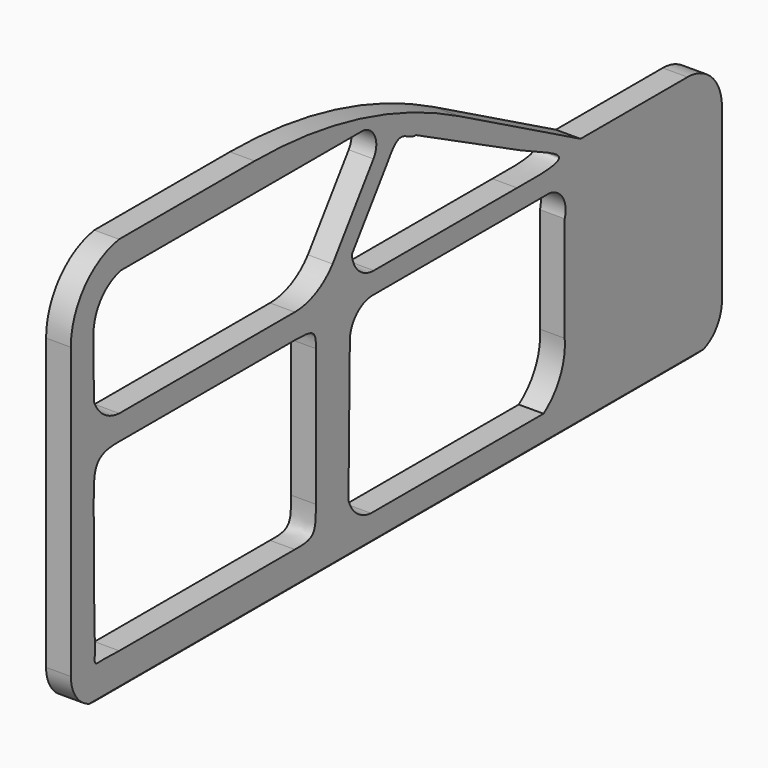
from build123d import *

# Parameters (mm, degrees)
F0_W     = 356.8245768547
F0_H     = 505.1945460796
F1_DEPTH = 50
F2_R     = 1088.3972766598
F3_R     = 86.9116882454
F4_SIZE  = 5
F5_R     = 72.4264068712


with BuildPart() as f1:
    # F0 (on Right) → F1 (new body)
    with BuildSketch(Plane.YZ):
        with BuildLine():
            Line((-202.2370483146, 445.1378583908), (-818.7412619591, 445.1378583908))
            ThreePointArc((-818.7412619591, 445.1378583908), (-905.8236422374, 396.3429239553), (-940.366268158, 302.6888072491))
            Line((-940.366268158, 302.6888072491), (-940.366268158, -354.9621416092))
            Line((-940.366268158, -354.9621416092), (345.9845781326, -354.9621416092))
            Line((345.9845781326, -354.9621416092), (345.9845781326, 150.2324044704))
            Line((345.9845781326, 150.2324044704), (-202.2370483146, 445.1378583908))
        make_face()
        with BuildLine():
            Line((-375.1508891582, -286.562114954), (-818.0344700813, -286.562114954))
            add(Edge.make_bspline(
                [(-881.003574872, -213.6291732903), (-872.4157214165, -310.1377487183), (-905.2422046661, -279.6560525894), (-818.0344700813, -286.562114954)],
                knots=[0, 0, 0, 0, 96.3551873946, 96.3551873946, 96.3551873946, 96.3551873946], degree=3))
            Line((-881.003574872, -213.6291732903), (-882.7309639931, 0))
            add(Edge.make_bspline(
                [(-882.7309639931, 0), (-883.1830024719, 63.9973655343), (-881.788790226, 86.3044932485), (-818.0344700813, 85.4378938675)],
                knots=[0, 0, 0, 0, 107.1693521161, 107.1693521161, 107.1693521161, 107.1693521161], degree=3))
            Line((-818.0344700813, 85.4378938675), (-375.1508891582, 85.4378938675))
            add(Edge.make_bspline(
                [(-375.1508891582, 85.4378938675), (-324.9171972275, 85.5383649468), (-321.6931819916, 79.6764940023), (-321.9781610433, 48.8521754742)],
                knots=[0, 0, 0, 0, 64.5434257345, 64.5434257345, 64.5434257345, 64.5434257345], degree=3))
            Line((-321.9781610433, 48.8521754742), (-321.9781610433, -227.8280258179))
            add(Edge.make_bspline(
                [(-375.1508891582, -286.562114954), (-320.8049535751, -288.4428203106), (-322.776645422, -274.6409773827), (-321.9781610433, -227.8280258179)],
                knots=[0, 0, 0, 0, 79.2277239471, 79.2277239471, 79.2277239471, 79.2277239471], degree=3))
        make_face(mode=Mode.SUBTRACT)
        with BuildLine():
            ThreePointArc((306.0723543167, -188.0455178505), (294.5381706361, -251.4470259438), (252.5045573711, -300.2933561802))
            Line((252.5045573711, -300.2933561802), (-182.7699840069, -300.2933561802))
            ThreePointArc((-182.7699840069, -300.2933561802), (-218.3948822871, -286.2867315588), (-239.6916596027, -254.4784592586))
            Line((-239.6916596027, -254.4784592586), (-236.269283319, 24.4449414313))
            ThreePointArc((-236.269283319, 24.4449414313), (-219.2164649006, 68.5667301116), (-175.0248968601, 85.4378938675))
            Line((-175.0248968601, 85.4378938675), (266.4457261562, 85.4378938675))
            ThreePointArc((266.4457261562, 85.4378938675), (300.8300474971, 64.4080832817), (306.0723543167, 24.4449414313))
            Line((306.0723543167, 24.4449414313), (306.0723543167, -188.0455178505))
        make_face(mode=Mode.SUBTRACT)
        with BuildLine():
            ThreePointArc((-883.216268158, 302.6888072501), (-863.6244382969, 357.7191784501), (-813.6645687377, 387.9878583908))
            Line((-813.6645687377, 387.9878583908), (-202.2370483146, 387.9878583908))
            ThreePointArc((-202.2370483146, 387.9878583908), (-172.4700911361, 364.5918803265), (-176.6405770461, 326.9614328601))
            Line((-176.6405770461, 326.9614328601), (-279.5936159166, 182.108691088))
            ThreePointArc((-279.5936159166, 182.108691088), (-321.9781610433, 147.7290262101), (-375.1508891582, 135.4378908872))
            Line((-375.1508891582, 135.4378908873), (-818.0344700841, 135.4378908873))
            ThreePointArc((-818.0344700841, 135.4378908873), (-857.2295081939, 149.4033105448), (-882.2456598282, 182.6520115127))
            Line((-882.2456598282, 182.6520115127), (-883.216268158, 302.6888072501))
        make_face(mode=Mode.SUBTRACT)
        with BuildLine():
            Line((-231.148657651, 179.4976291167), (-140.5107790807, 307.023201585))
            add(Edge.make_bspline(
                [(-140.5107790807, 307.023201585), (-106.8028062582, 362.7457022667), (-94.7402526246, 324.0503350315), (-69.5712245652, 325.77677484)],
                knots=[0, 0, 0, 0, 73.3765419238, 73.3765419238, 73.3765419238, 73.3765419238], degree=3))
            Line((-69.5712245652, 325.77677484), (194.9508041143, 191.1440640688))
            add(Edge.make_bspline(
                [(194.9508041143, 191.1440640688), (277.4597108364, 150.8727371693), (368.0824041367, 124.3830248713), (185.831874609, 128.1405687332)],
                knots=[0, 0, 0, 0, 63.6599976423, 63.6599976423, 63.6599976423, 63.6599976423], degree=3))
            Line((185.831874609, 128.1405687332), (-175.6092607975, 128.1405687332))
            ThreePointArc((-175.6092607975, 128.1405687332), (-213.4317813841, 142.9476106571), (-231.148657651, 179.4976291167))
        make_face(mode=Mode.SUBTRACT)
        with Locations((524.39686656, -102.3648685694)):
            Rectangle(F0_W, F0_H)
    extrude(amount=-F1_DEPTH)

    # F2
    f2_edges = [f1.edges().sort_by_distance(p)[0] for p in [
        (-25, -202.237048, 445.137858),
    ]]
    fillet(f2_edges, radius=F2_R)

    # F3
    f3_edges = [f1.edges().sort_by_distance(p)[0] for p in [
        (-25, 702.809155, 150.232404),
    ]]
    fillet(f3_edges, radius=F3_R)

    # F4
    f4_edges = [f1.edges().sort_by_distance(p)[0] for p in [
        (0, -118.778557, -354.962142),
        (-50, -118.778557, -354.962142),
    ]]
    chamfer(f4_edges, length=F4_SIZE)

    # F5
    f5_edges = [f1.edges().sort_by_distance(p)[0] for p in [
        (-25, 702.809155, -354.962142),
        (-25, -940.366268, -354.962142),
    ]]
    fillet(f5_edges, radius=F5_R)


solid = f1.part
